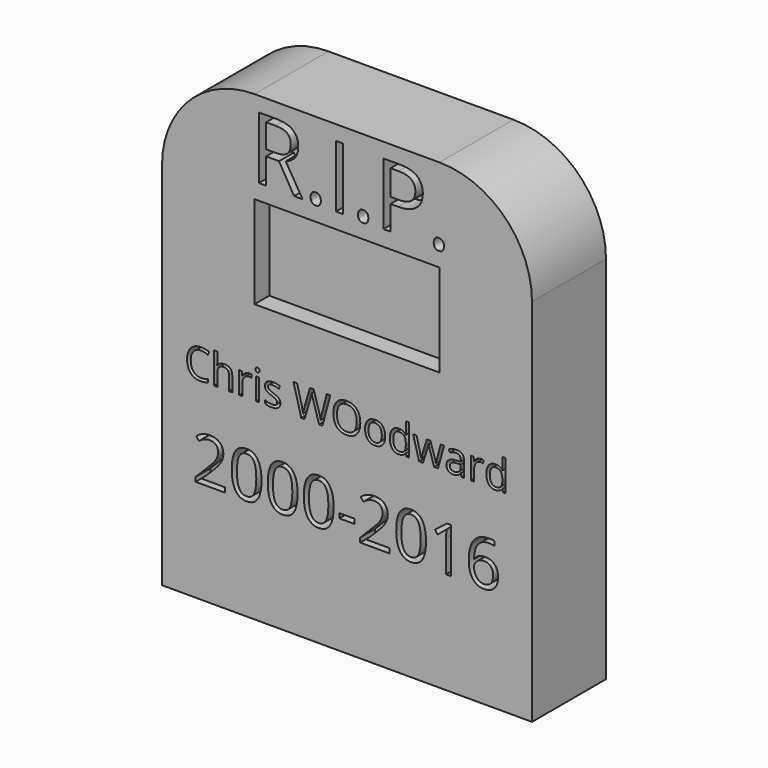
from build123d import *

# Parameters (mm, degrees)
F0_W           = 50.8
F0_H           = 25.4
F1_DEPTH       = 25.4
F2_DEPTH       = 20.32
F4_TEXT_SIZE   = 11.255836037
F4_TEXT_SIZE_2 = 17.3126735414
F5_DEPTH       = 5.08
F3_TEXT_SIZE   = 23.9318340189
F6_DEPTH       = 5.08


# Not quite as in the source:
# - Text() gives the source's letters only with a copy of the font that has no kerning and outlines rounded to 1/6400 em; it was checked with that copy


with BuildPart() as f1:
    # F0 (on Front) → F1 (new body)
    with BuildSketch(Plane.XZ):
        with BuildLine():
            Line((-46.1853042646, 40.2141681646), (-46.1853042646, -61.3858318354))
            Line((-46.1853042646, -61.3858318354), (55.4146957354, -61.3858318354))
            Line((55.4146957354, -61.3858318354), (55.4146957354, 40.2141681646))
            ThreePointArc((55.4146957354, 40.2141681646), (47.9752079776, 58.1746804067), (30.0146957354, 65.6141681646))
            Line((30.0146957354, 65.6141681646), (-20.7853042646, 65.6141681646))
            ThreePointArc((-20.7853042646, 65.6141681646), (-38.7458165067, 58.1746804067), (-46.1853042646, 40.2141681646))
        make_face()
        with Locations((4.6146957354, 27.5141681646)):
            Rectangle(F0_W, F0_H, mode=Mode.SUBTRACT)
    extrude(amount=F1_DEPTH)

    # F0 (on Front) → F2 (join)
    with BuildSketch(Plane.XZ):
        with Locations((4.6146957354, 27.5141681646)):
            Rectangle(F0_W, F0_H)
    extrude(amount=F2_DEPTH)

    # F4 (on face) → F5 (cut)
    with BuildSketch(Plane.XZ.offset(25.4)):
        with Locations((-39.9858439008, -8.4873492332)):
            Text('Chris WOodward', F4_TEXT_SIZE, font='Open Sans', text_align=(TextAlign.LEFT, TextAlign.BOTTOM))
        with Locations((-37.7954691648, -33.3789139986)):
            Text('2000-2016', F4_TEXT_SIZE_2, font='Open Sans', text_align=(TextAlign.LEFT, TextAlign.BOTTOM))
    extrude(amount=-F5_DEPTH, mode=Mode.SUBTRACT)

    # F3 (on face) → F6 (cut)
    with BuildSketch(Plane.XZ.offset(25.4)):
        with Locations((-21.9531208277, 44.4862581789)):
            Text('R.I.P.', F3_TEXT_SIZE, font='Open Sans', text_align=(TextAlign.LEFT, TextAlign.BOTTOM))
    extrude(amount=-F6_DEPTH, mode=Mode.SUBTRACT)


solid = f1.part
